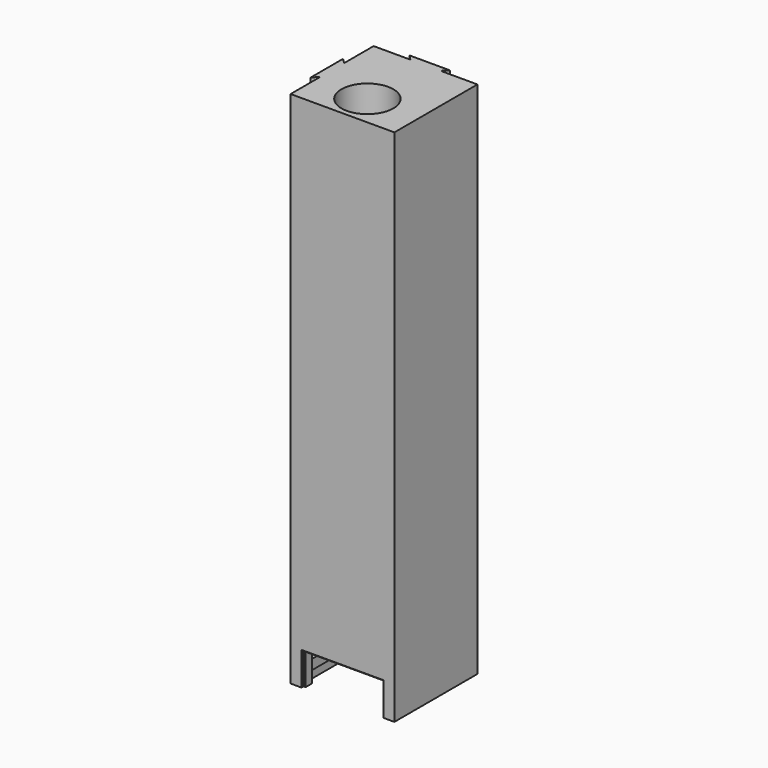
from build123d import *

# Parameters (mm, degrees)
F0_R     = 6.35
F1_DEPTH = 127
F2_R     = 6.35
F3_DEPTH = 7.62
F5_DEPTH = 0.635
F6_W     = 20.32
F6_H     = 2.413
F7_DEPTH = 1.016


# Not quite as in the source:
# - a feature names something its author has since deleted; it is built from what else it names


with BuildPart() as f1:
    # F0 (on Top) → F1 (new body)
    with BuildSketch(Plane.XY):
        Polygon((12.7, -12.7), (12.7, 12.7), (3.683, 12.7), (-3.683, 12.7), (-12.7, 12.7), (-12.7, 3.683), (-12.7, -3.683), (-12.7, -12.7), align=None)
        with Locations((0, -5.08)):
            Circle(F0_R, mode=Mode.SUBTRACT)
        Polygon((-13.97, -4.953), (-12.7, -3.683), (-12.7, 3.683), (-13.97, 4.953), align=None)
        Polygon((-3.683, 12.7), (3.683, 12.7), (4.953, 13.97), (-4.953, 13.97), align=None)
    extrude(amount=F1_DEPTH)

    # F2 (on face) → F3 (cut)
    with BuildSketch(Plane(origin=(0, 0, 0), x_dir=(1, 0, 0), z_dir=(0, 0, -1))):
        Polygon((9.525, 12.7), (-9.525, 12.7), (-9.525, 10.16), (-10.795, 10.16), (-10.795, -10.16), (10.795, -10.16), (10.795, 10.16), (9.525, 10.16), align=None)
        with Locations((0, 5.08)):
            Circle(F2_R, mode=Mode.SUBTRACT)
    extrude(amount=-F3_DEPTH, mode=Mode.SUBTRACT)

    # F4 (on face) → F5 (cut)
    with BuildSketch(Plane.XZ.offset(12.7)):
        Polygon((10.033, 8.128), (-10.033, 8.128), (-10.033, 0), (-9.525, 0), (-9.525, 7.62), (9.525, 7.62), (9.525, 0), (10.033, 0), align=None)
    extrude(amount=-F5_DEPTH, mode=Mode.SUBTRACT)



with BuildPart() as f7:
    # F6 (on face) → F7 (new body)
    with BuildSketch(Plane.YZ.offset(-10.795)):
        with Locations((0, 3.8735)):
            Rectangle(F6_W, F6_H)
    extrude(amount=F7_DEPTH)


with BuildPart() as f1_1:
    add(f1.part)

    add(f7.part)  # F8 merges F7
    # F8: F7 across plane
    add(f7.part.mirror(Plane.YZ))


with BuildPart() as f9_1:
    # F9: copy of F1
    add(f1_1.part)


solid = f1_1.part
